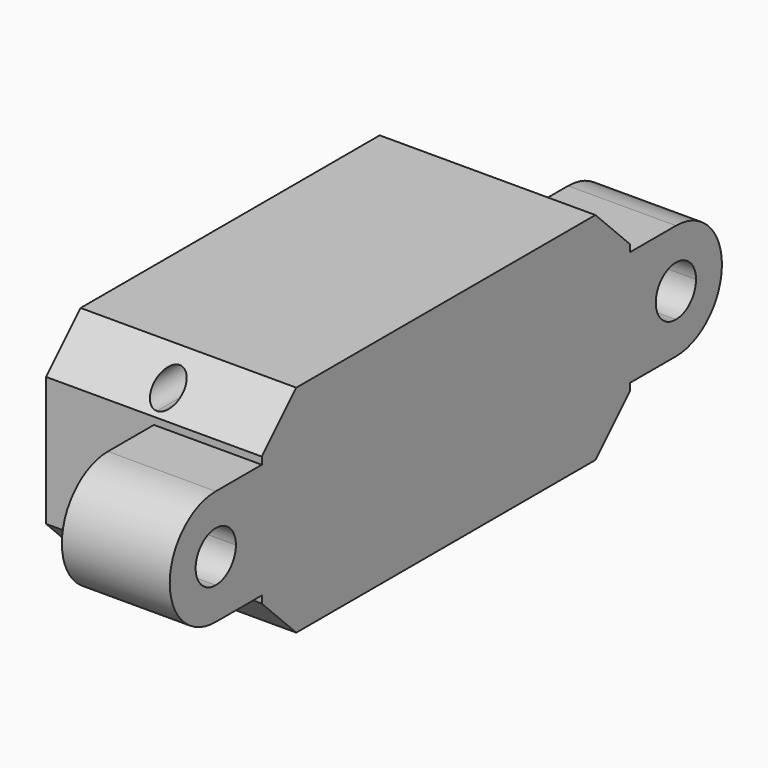
from build123d import *

# Parameters (mm, degrees)
F0_W        = 32
F0_H        = 3.5
F1_DEPTH    = 7.5
F2_DEPTH    = 7.5
F4_DEPTH    = 40
F5_T1_DEPTH = 30.4300979278


# Not quite as in the source:
# - a fillet or chamfer that OpenCascade refuses, or shapes differently, is made with other operations: its cross-section is extruded or revolved along the edge and cut away or added


with BuildPart() as f1:
    # F0 (on Right) → F1 (new body, symmetric)
    with BuildSketch(Plane.YZ):
        with Locations((0, -5.75)):
            Rectangle(F0_W, F0_H)
        Polygon((16, 0), (16, 4), (-16, 4), (-16, 0), (-16, -4), (16, -4), align=None)
        with Locations((0, 5.75)):
            Rectangle(F0_W, F0_H)
    extrude(amount=F1_DEPTH, both=True)

    # F0 (on Right) → F2 (join)
    with BuildSketch(Plane.YZ):
        with BuildLine():
            Line((-16, -4), (-16, 0))
            ThreePointArc((-16, 0), (-17.1715728753, -2.8284271247), (-20, -4))
            Line((-20, -4), (-16, -4))
        make_face()
        with BuildLine():
            ThreePointArc((-16, 0), (-17.1715728753, 2.8284271247), (-20, 4))
            Line((-20, 4), (-20, 1.75))
            ThreePointArc((-20, 1.75), (-18.7625631329, 1.2374368671), (-18.25, 0))
            ThreePointArc((-18.25, 0), (-18.7625631329, -1.2374368671), (-20, -1.75))
            Line((-20, -1.75), (-20, -4))
            ThreePointArc((-20, -4), (-17.1715728753, -2.8284271247), (-16, 0))
        make_face()
        with BuildLine():
            Line((-16, 0), (-16, 4))
            Line((-16, 4), (-20, 4))
            ThreePointArc((-20, 4), (-17.1715728753, 2.8284271247), (-16, 0))
        make_face()
        with BuildLine():
            Line((-20, 1.75), (-20, 4))
            ThreePointArc((-20, 4), (-24, 0), (-20, -4))
            Line((-20, -4), (-20, -1.75))
            ThreePointArc((-20, -1.75), (-21.75, 0), (-20, 1.75))
        make_face()
        with BuildLine():
            Line((20, 1.75), (20, 4))
            ThreePointArc((20, 4), (17.1715728753, 2.8284271247), (16, 0))
            ThreePointArc((16, 0), (17.1715728753, -2.8284271247), (20, -4))
            Line((20, -4), (20, -1.75))
            ThreePointArc((20, -1.75), (18.25, 0), (20, 1.75))
        make_face()
        with BuildLine():
            ThreePointArc((16, 0), (17.1715728753, 2.8284271247), (20, 4))
            Line((20, 4), (16, 4))
            Line((16, 4), (16, 0))
        make_face()
        with BuildLine():
            ThreePointArc((20, -4), (17.1715728753, -2.8284271247), (16, 0))
            Line((16, 0), (16, -4))
            Line((16, -4), (20, -4))
        make_face()
        with BuildLine():
            ThreePointArc((24, 0), (22.8284271247, 2.8284271247), (20, 4))
            Line((20, 4), (20, 1.75))
            ThreePointArc((20, 1.75), (21.2374368671, 1.2374368671), (21.75, 0))
            ThreePointArc((21.75, 0), (21.2374368671, -1.2374368671), (20, -1.75))
            Line((20, -1.75), (20, -4))
            ThreePointArc((20, -4), (22.8284271247, -2.8284271247), (24, 0))
        make_face()
    extrude(amount=F2_DEPTH)

    # F3 (on face) → F4 (cut)
    with BuildSketch(Plane.XZ.offset(16)):
        with BuildLine():
            ThreePointArc((1, 5.75), (0.7071067812, 6.4571067812), (0, 6.75))
            Line((0, 6.75), (0, 4.75))
            ThreePointArc((0, 4.75), (0.7071067812, 5.0428932188), (1, 5.75))
        make_face()
        with BuildLine():
            Line((0, 4.75), (0, 6.75))
            ThreePointArc((0, 6.75), (-1, 5.75), (0, 4.75))
        make_face()
        with BuildLine():
            ThreePointArc((1, -5.75), (0.7071067812, -5.0428932188), (0, -4.75))
            Line((0, -4.75), (0, -6.75))
            ThreePointArc((0, -6.75), (0.7071067812, -6.4571067812), (1, -5.75))
        make_face()
        with BuildLine():
            Line((0, -6.75), (0, -4.75))
            ThreePointArc((0, -4.75), (-1, -5.75), (0, -6.75))
        make_face()
    extrude(amount=-F4_DEPTH, mode=Mode.SUBTRACT)

    # F5: chamfer of 3 on 4 edges, made by hand

    # F5_s2 → F5_t1 (cut)
    with BuildSketch(Plane.YZ.offset(-15.2150489639)):
        Polygon((-13, 7.5), (-16, 4.5), (-16, 7.5), align=None)
        Polygon((-13, -7.5), (-16, -4.5), (-16, -7.5), align=None)
        Polygon((16, 4.5), (13, 7.5), (16, 7.5), align=None)
        Polygon((16, -4.5), (13, -7.5), (16, -7.5), align=None)
    extrude(amount=F5_T1_DEPTH, mode=Mode.SUBTRACT)


solid = f1.part
